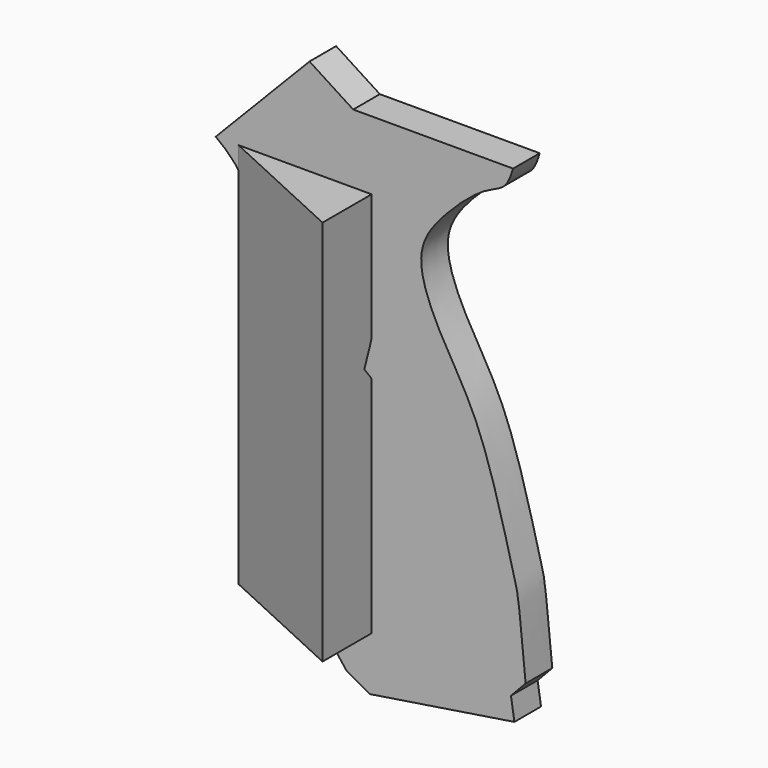
from build123d import *

# Parameters (mm, degrees)
F1_DEPTH = 9.525


with BuildPart() as f1:
    # F0 (on Front) → F1 (new body)
    with BuildSketch(Plane.XZ):
        with BuildLine():
            Line((25.5529873787, 2.8441333306), (-20.1670126213, 2.8441333306))
            Line((-20.1670126213, 2.8441333306), (-32.6776243746, 10.8811762184))
            Line((-32.6776243746, 10.8811762184), (-59.5039837062, -16.7887844145))
            ThreePointArc((-59.5039837062, -16.7887844145), (-47.1561716454, -36.685361085), (-53.0086271465, -59.3589358032))
            ThreePointArc((-53.0086271465, -59.3589358032), (-43.8175889792, -73.3576679015), (-42.0523360372, -90.01070261))
            ThreePointArc((-42.0523360372, -90.01070261), (-32.7557600238, -107.5361024576), (-31.236698851, -127.3163557053))
            Line((-31.236698851, -127.3163557053), (-21.9750162214, -139.2256170511))
            Line((-21.9750162214, -139.2256170511), (-15.3611972928, -142.8006440401))
            Line((-15.3611972928, -142.8006440401), (25.9304773062, -136.3655775785))
            Line((25.9304773062, -136.3655775785), (24.9513892664, -130.0830962729))
            Line((24.9513892664, -130.0830962729), (29.148010537, -125.6404668093))
            add(Edge.make_bspline(
                [(29.148010537, -125.6404668093), (28.2946798198, -116.6393923055), (27.0527948496, -103.5397828384), (25.6464249734, -99.678769998), (17.4501539035, -65.5456126073), (6.0747879382, -48.5212865138), (-0.6953024195, -34.3483750512), (-1.2258021041, -23.7384798264), (6.8210480205, -13.805998052), (17.0170487732, -4.8279874656), (23.6734646695, -3.1092179724), (24.9350590303, 0.8868574115), (25.5529873787, 2.8441333306)],
                knots=[0, 0, 0, 0, 0.1286807075, 0.1872739764, 0.3453426722, 0.476808041, 0.5820736122, 0.6673622055, 0.7644318863, 0.8660039058, 0.9343687735, 1, 1, 1, 1], degree=3))
        make_face()
    extrude(amount=F1_DEPTH)


with BuildPart() as f6:
    # F5 (on face) → F6 section 0
    with BuildSketch(Plane.YZ.offset(-14.9086271465)):
        with BuildLine():
            ThreePointArc((-12.1535348742, -59.8138779625), (-6.7159535078, -38.5900093867), (-8.89, -16.7887844145))
            Line((-8.89, -16.7887844145), (-27.0782951266, -16.7887844145))
            Line((-27.0782951266, -16.7887844145), (-27.0782951266, -127.3163557053))
            Line((-27.0782951266, -127.3163557053), (-6.35, -127.3163557053))
            ThreePointArc((-6.35, -127.3163557053), (-3.7730338417, -108.0780656946), (-6.6773612612, -88.8864675498))
            ThreePointArc((-6.6773612612, -88.8864675498), (-5.4089924739, -73.595508424), (-12.1535348742, -59.8138779625))
        make_face()
    # F3 (on face) → F6 section 1
    with BuildSketch(Plane.YZ.offset(-53.0086271465)):
        with BuildLine():
            Line((-2.54, -16.7887844145), (-9.525, -16.7887844145))
            Line((-9.525, -16.7887844145), (-9.525, -127.3163557053))
            Line((-9.525, -127.3163557053), (-5.08, -127.3163557053))
            ThreePointArc((-5.08, -127.3163557053), (-2.8796392632, -108.6635291576), (-5.08, -90.01070261))
            ThreePointArc((-5.08, -90.01070261), (-2.0522838803, -74.6848192066), (-5.08, -59.3589358032))
            ThreePointArc((-5.08, -59.3589358032), (-0.6907278213, -38.2599752876), (-2.54, -16.7887844145))
        make_face()
    loft()


solid = Compound([f1.part, f6.part])
